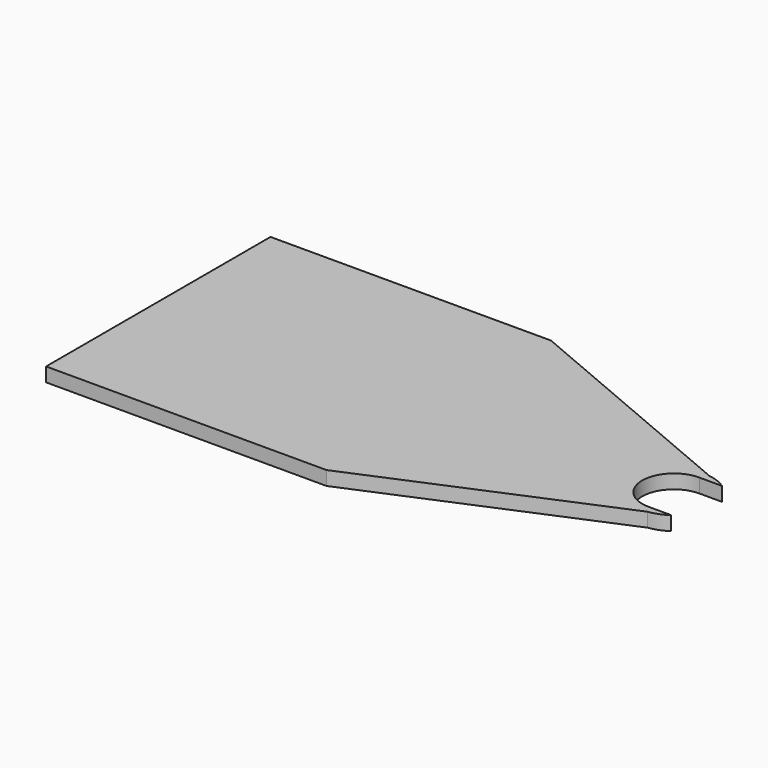
from build123d import *

# Parameters (mm, degrees)
F0_W     = 54
F0_H     = 54
F1_DEPTH = 2.7


# Not quite as in the source:
# - a feature names something its author has since deleted; it is built from what else it names


with BuildPart() as f1:
    # F0 (on Top) → F1 (new body)
    with BuildSketch(Plane.XY):
        with Locations((-60.3654519308, -7.9408198703)):
            Rectangle(F0_W, F0_H)
        with BuildLine():
            Line((-33.3654519308, -34.9408198703), (12.8123124507, -15.3844278592))
            ThreePointArc((12.8123124507, -15.3844278592), (14.6191753291, -14.9283225153), (16.2578103101, -14.0408198703))
            Line((16.2578103101, -14.0408198703), (11.8943254642, -14.0408198703))
            ThreePointArc((11.8943254642, -14.0408198703), (5.7943254642, -7.9408198703), (11.8943254642, -1.8408198703))
            Line((11.8943254642, -1.8408198703), (16.2578103101, -1.8408198703))
            ThreePointArc((16.2578103101, -1.8408198703), (14.6191753291, -0.9533172253), (12.8123124507, -0.4972118814))
            Line((12.8123124507, -0.4972118814), (-33.3654519308, 19.0591801297))
            Line((-33.3654519308, 19.0591801297), (-33.3654519308, -34.9408198703))
        make_face()
    extrude(amount=F1_DEPTH)


solid = f1.part
